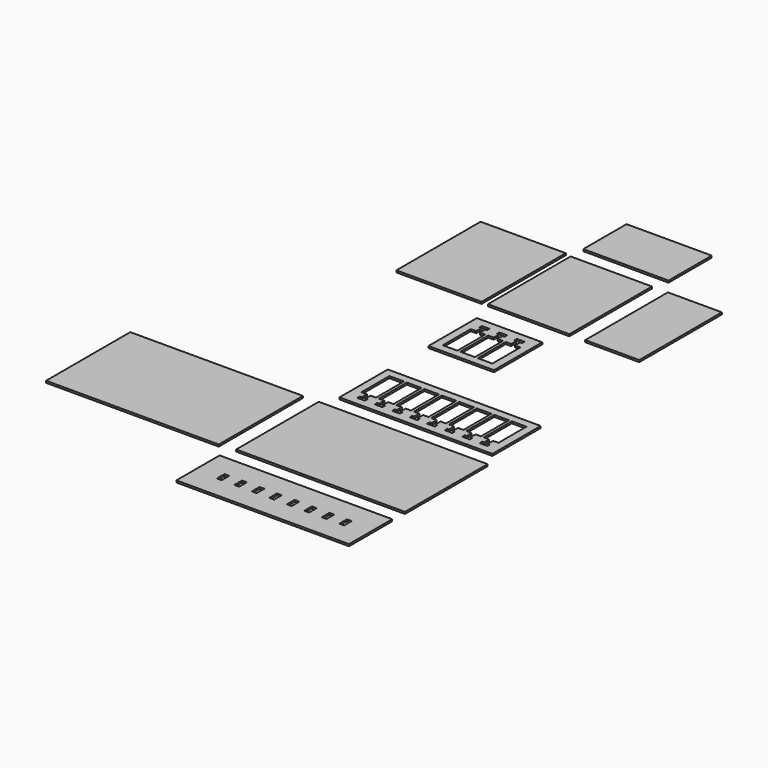
from build123d import *

# Parameters (mm, degrees)
F0_W     = 481
F0_H     = 190
F1_DEPTH = 6
F0_W_2   = 206
F0_W_3   = 531
F0_H_2   = 325
F2_DEPTH = 6
F0_W_4   = 256
F0_W_5   = 170
F0_W_6   = 268
F0_H_3   = 170
F0_H_4   = 331
F0_W_7   = 543
F0_W_8   = 15
F0_H_5   = 30


# Not quite as in the source:
# - a feature names something its author has since deleted; it is built from what else it names


with BuildPart() as f1:
    # F0 (on Top) → F1 (new body)
    with BuildSketch(Plane.XY):
        with Locations((215.5, 40)):
            Rectangle(F0_W, F0_H)
        Polygon((17, 0), (0, 0), (0, 110), (46, 110), (46, 0), (29, 0), (29, -20), (35, -20), (35, -30), (29, -30), (17, -30), (11, -30), (11, -20), (17, -20), align=None, mode=Mode.SUBTRACT)
        Polygon((101, 110), (101, 0), (84, 0), (84, -20), (90, -20), (90, -30), (84, -30), (72, -30), (66, -30), (66, -20), (72, -20), (72, 0), (55, 0), (55, 110), align=None, mode=Mode.SUBTRACT)
        Polygon((156, 110), (156, 0), (139, 0), (139, -20), (145, -20), (145, -30), (139, -30), (127, -30), (121, -30), (121, -20), (127, -20), (127, 0), (110, 0), (110, 110), align=None, mode=Mode.SUBTRACT)
        Polygon((211, 110), (211, 0), (194, 0), (194, -20), (200, -20), (200, -30), (194, -30), (182, -30), (176, -30), (176, -20), (182, -20), (182, 0), (165, 0), (165, 110), align=None, mode=Mode.SUBTRACT)
        Polygon((266, 110), (266, 0), (249, 0), (249, -20), (255, -20), (255, -30), (249, -30), (237, -30), (231, -30), (231, -20), (237, -20), (237, 0), (220, 0), (220, 110), align=None, mode=Mode.SUBTRACT)
        Polygon((321, 110), (321, 0), (304, 0), (304, -20), (310, -20), (310, -30), (304, -30), (292, -30), (286, -30), (286, -20), (292, -20), (292, 0), (275, 0), (275, 110), align=None, mode=Mode.SUBTRACT)
        Polygon((376, 110), (376, 0), (359, 0), (359, -20), (365, -20), (365, -30), (359, -30), (347, -30), (341, -30), (341, -20), (347, -20), (347, 0), (330, 0), (330, 110), align=None, mode=Mode.SUBTRACT)
        Polygon((431, 110), (431, 0), (414, 0), (414, -20), (420, -20), (420, -30), (414, -30), (402, -30), (396, -30), (396, -20), (402, -20), (402, 0), (385, 0), (385, 110), align=None, mode=Mode.SUBTRACT)
    extrude(amount=F1_DEPTH)


with BuildPart() as f1b:
    # F0 (on Top) → F1, piece 2 (new body)
    with BuildSketch(Plane.XY):
        with Locations((78, 390)):
            Rectangle(F0_W_2, F0_H)
        Polygon((17, 430), (17, 450), (11, 450), (11, 460), (17, 460), (29, 460), (35, 460), (35, 450), (29, 450), (29, 430), (46, 430), (46, 320), (0, 320), (0, 430), align=None, mode=Mode.SUBTRACT)
        Polygon((72, 460), (84, 460), (90, 460), (90, 450), (84, 450), (84, 430), (101, 430), (101, 320), (55, 320), (55, 430), (72, 430), (72, 450), (66, 450), (66, 460), align=None, mode=Mode.SUBTRACT)
        Polygon((127, 460), (139, 460), (145, 460), (145, 450), (139, 450), (139, 430), (156, 430), (156, 320), (110, 320), (110, 430), (127, 430), (127, 450), (121, 450), (121, 460), align=None, mode=Mode.SUBTRACT)
    extrude(amount=F1_DEPTH)


with BuildPart() as f2:
    # F0 (on Top) → F2 (new body)
    with BuildSketch(Plane.XY):
        with Locations((215.5, -267.5)):
            Rectangle(F0_W_3, F0_H_2)
    extrude(amount=F2_DEPTH)


with BuildPart() as f2b:
    # F0 (on Top) → F2, piece 2 (new body)
    with BuildSketch(Plane.XY):
        with Locations((78, 722.5)):
            Rectangle(F0_W_4, F0_H_2)
    extrude(amount=F2_DEPTH)


with BuildPart() as f2c:
    # F0 (on Top) → F2, piece 3 (new body)
    with BuildSketch(Plane.XY):
        with Locations((341, 722.5)):
            Rectangle(F0_W_5, F0_H_2)
    extrude(amount=F2_DEPTH)


with BuildPart() as f2d:
    # F0 (on Top) → F2, piece 4 (new body)
    with BuildSketch(Plane.XY):
        with Locations((84, 1020)):
            Rectangle(F0_W_6, F0_H_3)
    extrude(amount=F2_DEPTH)


with BuildPart() as f2e:
    # F0 (on Top) → F2, piece 5 (new body)
    with BuildSketch(Plane.XY):
        with Locations((-204, 725.5)):
            Rectangle(F0_W_6, F0_H_4)
    extrude(amount=F2_DEPTH)


with BuildPart() as f2f:
    # F0 (on Top) → F2, piece 6 (new body)
    with BuildSketch(Plane.XY):
        with Locations((209.5, -565)):
            Rectangle(F0_W_7, F0_H_3)
        with Locations((17, -565)):
            Rectangle(F0_W_8, F0_H_5, mode=Mode.SUBTRACT)
        with Locations((72, -565)):
            Rectangle(F0_W_8, F0_H_5, mode=Mode.SUBTRACT)
        with Locations((127, -565)):
            Rectangle(F0_W_8, F0_H_5, mode=Mode.SUBTRACT)
        with Locations((182, -565)):
            Rectangle(F0_W_8, F0_H_5, mode=Mode.SUBTRACT)
        with Locations((237, -565)):
            Rectangle(F0_W_8, F0_H_5, mode=Mode.SUBTRACT)
        with Locations((292, -565)):
            Rectangle(F0_W_8, F0_H_5, mode=Mode.SUBTRACT)
        with Locations((347, -565)):
            Rectangle(F0_W_8, F0_H_5, mode=Mode.SUBTRACT)
        with Locations((402, -565)):
            Rectangle(F0_W_8, F0_H_5, mode=Mode.SUBTRACT)
    extrude(amount=F2_DEPTH)


with BuildPart() as f2g:
    # F0 (on Top) → F2, piece 7 (new body)
    with BuildSketch(Plane.XY):
        with Locations((-371.5, -270.5)):
            Rectangle(F0_W_7, F0_H_4)
    extrude(amount=F2_DEPTH)


solid = Compound([f1.part, f1b.part, f2.part, f2b.part, f2c.part, f2d.part, f2e.part, f2f.part, f2g.part])
